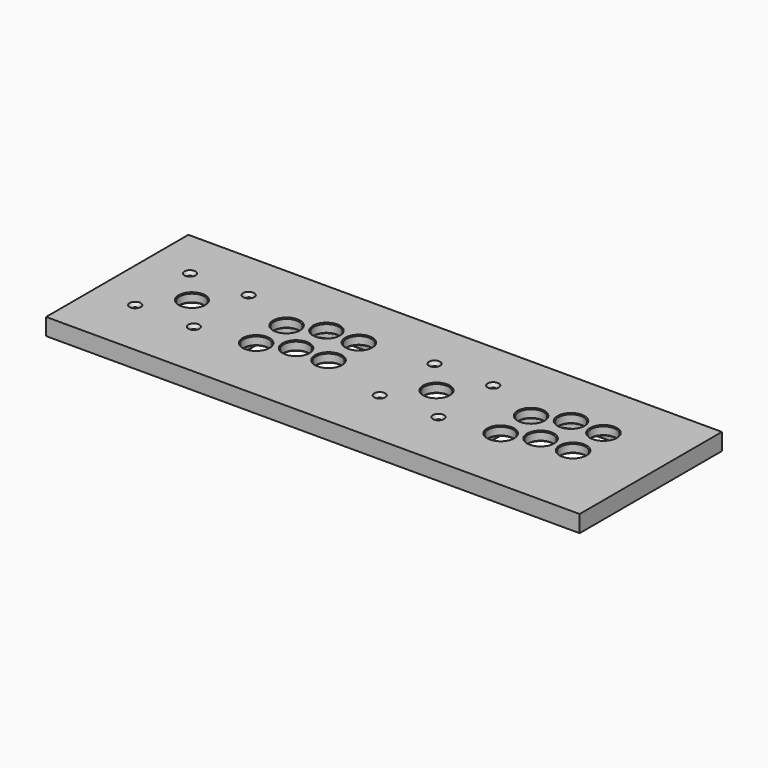
from build123d import *

# Parameters (mm, degrees)
F0_W     = 600
F0_H     = 200
F0_R     = 14.2
F0_R_2   = 14
F1_DEPTH = 19
F2_R     = 14.2
F2_W     = 79.5
F2_H     = 96.5
F2_R_2   = 2.75
F2_R_3   = 14
F3_DEPTH = 8.5
F4_DEPTH = 19.001
F5_R     = 5
F6_SIZE  = 3.5
F7_SIZE  = 1


# Not quite as in the source:
# - a feature names something its author has since deleted; it is built from what else it names


with BuildPart() as f1:
    # F0 (on Top) → F1 (new body)
    with BuildSketch(Plane.XY):
        Rectangle(F0_W, F0_H)
        with Locations((-125, -23.5)):
            Circle(F0_R, mode=Mode.SUBTRACT)
        with Locations((-91.5, -9.25)):
            Circle(F0_R, mode=Mode.SUBTRACT)
        with Locations((-55, -9.25)):
            Circle(F0_R, mode=Mode.SUBTRACT)
        with Locations((150, -23.5)):
            Circle(F0_R, mode=Mode.SUBTRACT)
        with Locations((183.5, -9.25)):
            Circle(F0_R, mode=Mode.SUBTRACT)
        with Locations((220, -9.25)):
            Circle(F0_R, mode=Mode.SUBTRACT)
        with Locations((-220, 5)):
            Circle(F0_R_2, mode=Mode.SUBTRACT)
        with Locations((-125, 19.25)):
            Circle(F0_R, mode=Mode.SUBTRACT)
        with Locations((-91.5, 33.5)):
            Circle(F0_R, mode=Mode.SUBTRACT)
        with Locations((-55, 33.5)):
            Circle(F0_R, mode=Mode.SUBTRACT)
        with Locations((55, 5)):
            Circle(F0_R_2, mode=Mode.SUBTRACT)
        with Locations((150, 19.25)):
            Circle(F0_R, mode=Mode.SUBTRACT)
        with Locations((183.5, 33.5)):
            Circle(F0_R, mode=Mode.SUBTRACT)
        with Locations((220, 33.5)):
            Circle(F0_R, mode=Mode.SUBTRACT)
    extrude(amount=F1_DEPTH)

    # F2 (on face) → F3 (cut)
    with BuildSketch(Plane(origin=(0, 0, 0), x_dir=(1, 0, 0), z_dir=(0, 0, -1))):
        with BuildLine():
            ThreePointArc((-98.9371975615, -50.9839381271), (-95.2950741485, -52.1171268516), (-91.5, -52.5))
            Line((-91.5, -52.5), (-55, -52.5))
            ThreePointArc((-55, -52.5), (-41.5649711575, -46.9350288425), (-36, -33.5))
            Line((-36, -33.5), (-36, 9.25))
            ThreePointArc((-36, 9.25), (-41.5649711575, 22.6850288425), (-55, 28.25))
            ThreePointArc((-55, 28.25), (-86.9227874299, 31.4657900344), (-117.5628024385, 40.9839381271))
            ThreePointArc((-117.5628024385, 40.9839381271), (-135.4807739774, 39.3478193085), (-144, 23.5))
            Line((-144, 23.5), (-144, -19.25))
            ThreePointArc((-144, -19.25), (-140.8478193085, -29.7307739774), (-132.4371975615, -36.7339381271))
            Line((-132.4371975615, -36.7339381271), (-98.9371975615, -50.9839381271))
        make_face()
        with Locations((-91.5, -33.5)):
            Circle(F2_R, mode=Mode.SUBTRACT)
        with Locations((-55, -33.5)):
            Circle(F2_R, mode=Mode.SUBTRACT)
        with Locations((-125, -19.25)):
            Circle(F2_R, mode=Mode.SUBTRACT)
        with Locations((-91.5, 9.25)):
            Circle(F2_R, mode=Mode.SUBTRACT)
        with Locations((-125, 23.5)):
            Circle(F2_R, mode=Mode.SUBTRACT)
        with Locations((-55, 9.25)):
            Circle(F2_R, mode=Mode.SUBTRACT)
        with BuildLine():
            ThreePointArc((131, -19.25), (134.1521806915, -29.7307739774), (142.5628024385, -36.7339381271))
            Line((142.5628024385, -36.7339381271), (176.0628024385, -50.9839381271))
            ThreePointArc((176.0628024385, -50.9839381271), (179.7049258515, -52.1171268516), (183.5, -52.5))
            Line((183.5, -52.5), (220, -52.5))
            ThreePointArc((220, -52.5), (233.4350288425, -46.9350288425), (239, -33.5))
            Line((239, -33.5), (239, 9.25))
            ThreePointArc((239, 9.25), (233.4350288425, 22.6850288425), (220, 28.25))
            ThreePointArc((220, 28.25), (188.0772125701, 31.4657900344), (157.4371975615, 40.9839381271))
            ThreePointArc((157.4371975615, 40.9839381271), (139.5192260226, 39.3478193085), (131, 23.5))
            Line((131, 23.5), (131, -19.25))
        make_face()
        with Locations((183.5, -33.5)):
            Circle(F2_R, mode=Mode.SUBTRACT)
        with Locations((220, -33.5)):
            Circle(F2_R, mode=Mode.SUBTRACT)
        with Locations((150, -19.25)):
            Circle(F2_R, mode=Mode.SUBTRACT)
        with Locations((183.5, 9.25)):
            Circle(F2_R, mode=Mode.SUBTRACT)
        with Locations((220, 9.25)):
            Circle(F2_R, mode=Mode.SUBTRACT)
        with Locations((150, 23.5)):
            Circle(F2_R, mode=Mode.SUBTRACT)
        with Locations((-220, -5)):
            Rectangle(F2_W, F2_H)
        with Locations((-253, -43.5)):
            Circle(F2_R_2, mode=Mode.SUBTRACT)
        with Locations((-187, -43.5)):
            Circle(F2_R_2, mode=Mode.SUBTRACT)
        with Locations((-220, -5)):
            Circle(F2_R_3, mode=Mode.SUBTRACT)
        with Locations((-253, 33.5)):
            Circle(F2_R_2, mode=Mode.SUBTRACT)
        with Locations((-187, 33.5)):
            Circle(F2_R_2, mode=Mode.SUBTRACT)
        with Locations((55, -5)):
            Rectangle(F2_W, F2_H)
        with Locations((22, -43.5)):
            Circle(F2_R_2, mode=Mode.SUBTRACT)
        with Locations((88, -43.5)):
            Circle(F2_R_2, mode=Mode.SUBTRACT)
        with Locations((55, -5)):
            Circle(F2_R_3, mode=Mode.SUBTRACT)
        with Locations((22, 33.5)):
            Circle(F2_R_2, mode=Mode.SUBTRACT)
        with Locations((88, 33.5)):
            Circle(F2_R_2, mode=Mode.SUBTRACT)
        with Locations((-253, 33.5)):
            Circle(F2_R_2)
        with Locations((-187, 33.5)):
            Circle(F2_R_2)
        with Locations((-187, -43.5)):
            Circle(F2_R_2)
        with Locations((-253, -43.5)):
            Circle(F2_R_2)
        with Locations((22, 33.5)):
            Circle(F2_R_2)
        with Locations((88, 33.5)):
            Circle(F2_R_2)
        with Locations((88, -43.5)):
            Circle(F2_R_2)
        with Locations((22, -43.5)):
            Circle(F2_R_2)
    extrude(amount=-F3_DEPTH, mode=Mode.SUBTRACT)

    # F2 (on face) → F4 (cut, through all)
    with BuildSketch(Plane(origin=(0, 0, 0), x_dir=(1, 0, 0), z_dir=(0, 0, -1))):
        with Locations((-253, 33.5)):
            Circle(F2_R_2)
        with Locations((-187, 33.5)):
            Circle(F2_R_2)
        with Locations((-187, -43.5)):
            Circle(F2_R_2)
        with Locations((-253, -43.5)):
            Circle(F2_R_2)
        with Locations((22, 33.5)):
            Circle(F2_R_2)
        with Locations((88, 33.5)):
            Circle(F2_R_2)
        with Locations((88, -43.5)):
            Circle(F2_R_2)
        with Locations((22, -43.5)):
            Circle(F2_R_2)
    extrude(amount=-F4_DEPTH, mode=Mode.SUBTRACT)

    # F5
    f5_edges = [f1.edges().sort_by_distance(p)[0] for p in [
        (-259.75, -43.25, 4.25),
        (-180.25, -43.25, 4.25),
        (-180.25, 53.25, 4.25),
        (-259.75, 53.25, 4.25),
        (15.25, 53.25, 4.25),
        (15.25, -43.25, 4.25),
        (94.75, -43.25, 4.25),
        (94.75, 53.25, 4.25),
    ]]
    fillet(f5_edges, radius=F5_R)

    # F6
    f6_edges = [f1.edges().sort_by_distance(p)[0] for p in [
        (85.25, -33.5, 19),
        (85.25, 43.5, 19),
        (19.25, 43.5, 19),
        (19.25, -33.5, 19),
        (-189.75, 43.5, 19),
        (-189.75, -33.5, 19),
        (-255.75, -33.5, 19),
        (-255.75, 43.5, 19),
    ]]
    chamfer(f6_edges, length=F6_SIZE)

    # F7
    f7_edges = [f1.edges().sort_by_distance(p)[0] for p in [
        (-234, 5, 8.5),
        (-206, 5, 13.75),
        (-234, 5, 19),
        (-139.2, 19.25, 8.5),
        (-110.8, 19.25, 13.75),
        (-139.2, 19.25, 19),
        (-105.7, 33.5, 8.5),
        (-77.3, 33.5, 13.75),
        (-105.7, 33.5, 19),
        (-139.2, -23.5, 8.5),
        (-110.8, -23.5, 13.75),
        (-139.2, -23.5, 19),
        (-105.7, -9.25, 8.5),
        (-77.3, -9.25, 13.75),
        (-105.7, -9.25, 19),
        (-69.2, -9.25, 8.5),
        (-40.8, -9.25, 13.75),
        (-69.2, -9.25, 19),
        (-69.2, 33.5, 8.5),
        (-40.8, 33.5, 13.75),
        (-69.2, 33.5, 19),
        (41, 5, 8.5),
        (69, 5, 13.75),
        (41, 5, 19),
        (135.8, 19.25, 8.5),
        (164.2, 19.25, 13.75),
        (135.8, 19.25, 19),
        (135.8, -23.5, 8.5),
        (164.2, -23.5, 13.75),
        (135.8, -23.5, 19),
        (169.3, -9.25, 8.5),
        (197.7, -9.25, 13.75),
        (169.3, -9.25, 19),
        (169.3, 33.5, 8.5),
        (197.7, 33.5, 13.75),
        (169.3, 33.5, 19),
        (205.8, 33.5, 8.5),
        (234.2, 33.5, 13.75),
        (205.8, 33.5, 19),
        (205.8, -9.25, 8.5),
        (234.2, -9.25, 13.75),
        (205.8, -9.25, 19),
        (55, 53.25, 0),
        (-220, 53.25, 0),
        (-86.922787, -31.46579, 0),
        (188.077213, -31.46579, 0),
    ]]
    chamfer(f7_edges, length=F7_SIZE)


solid = f1.part
